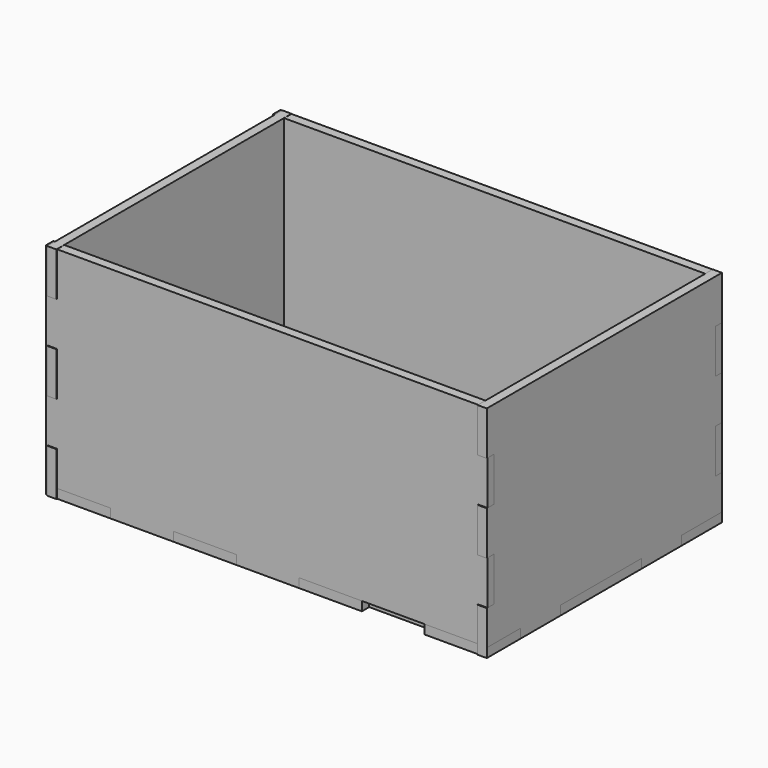
from build123d import *

# Parameters (mm, degrees)
F0_W     = 18.5964285714
F0_H     = 3.175
F0_W_2   = 3.175
F0_H_2   = 14.2994610153
F0_H_3   = 17.4744610153
F0_H_4   = 11.0526949236
F0_W_3   = 21.7714285714
F1_DEPTH = 3.175
F2_W     = 3.175
F2_H     = 15.24
F2_W_2   = 2.8866035402
F3_DEPTH = 3.175
F6_DEPTH = 3.175


with BuildPart() as f1:
    # F0 (on Top) → F1 (new body)
    with BuildSketch(Plane.XY):
        with Locations((-63.7267857143, 49.2125)):
            Rectangle(F0_W, F0_H)
        with Locations((-74.6125, 49.2125)):
            Rectangle(F0_W_2, F0_H)
        with Locations((-74.6125, 40.4752694924)):
            Rectangle(F0_W_2, F0_H_2)
        with Locations((-74.6125, 7.1138474618)):
            Rectangle(F0_W_2, F0_H_3)
        with Locations((-74.6125, -10.3606135535)):
            Rectangle(F0_W_2, F0_H_3)
        with Locations((-74.6125, -42.0986525382)):
            Rectangle(F0_W_2, F0_H_4)
        with Locations((-74.6125, -49.2125)):
            Rectangle(F0_W_2, F0_H)
        with Locations((-63.7267857143, -49.2125)):
            Rectangle(F0_W, F0_H)
        with Locations((-21.7714285714, -49.2125)):
            Rectangle(F0_W_3, F0_H)
        with Locations((21.7714285714, -49.2125)):
            Rectangle(F0_W_3, F0_H)
        with Locations((63.7267857143, -49.2125)):
            Rectangle(F0_W, F0_H)
        with Locations((74.6125, -42.0986525382)):
            Rectangle(F0_W_2, F0_H_4)
        with Locations((74.6125, -10.3606135535)):
            Rectangle(F0_W_2, F0_H_3)
        with Locations((74.6125, 7.1138474618)):
            Rectangle(F0_W_2, F0_H_3)
        with Locations((74.6125, 40.4752694924)):
            Rectangle(F0_W_2, F0_H_2)
        with Locations((74.6125, 49.2125)):
            Rectangle(F0_W_2, F0_H)
        with Locations((63.7267857143, 49.2125)):
            Rectangle(F0_W, F0_H)
        with Locations((21.7714285714, 49.2125)):
            Rectangle(F0_W_3, F0_H)
        with Locations((-21.7714285714, 49.2125)):
            Rectangle(F0_W_3, F0_H)
        Polygon((73.025, 33.3255389847), (73.025, 47.625), (54.4285714286, 47.625), (32.6571428571, 47.625), (10.8857142857, 47.625), (-10.8857142857, 47.625), (-32.6571428571, 47.625), (-54.4285714286, 47.625), (-73.025, 47.625), (-73.025, 33.3255389847), (-73.025, 15.8510779694), (-73.025, -1.6233830458), (-73.025, -19.0978440611), (-73.025, -36.5723050764), (-73.025, -47.625), (-54.4285714286, -47.625), (-32.6571428571, -47.625), (-10.8857142857, -47.625), (10.8857142857, -47.625), (32.6571428571, -47.625), (54.4285714286, -47.625), (73.025, -47.625), (73.025, -36.5723050764), (73.025, -19.0978440611), (73.025, -1.6233830458), (73.025, 15.8510779694), align=None)
    extrude(amount=F1_DEPTH)

    # F2 (on face) → F3 (join)
    with BuildSketch(Plane.YZ.offset(76.2)):
        with Locations((-49.5008964598, 68.58)):
            Rectangle(F2_W, F2_H)
        with Locations((-49.5008964598, 38.1)):
            Rectangle(F2_W, F2_H)
        with Locations((-49.5008964598, 7.62)):
            Rectangle(F2_W, F2_H)
        with Locations((49.3566982299, 38.1)):
            Rectangle(F2_W_2, F2_H)
        with Locations((49.3566982299, 7.62)):
            Rectangle(F2_W_2, F2_H)
        with Locations((49.3566982299, 68.58)):
            Rectangle(F2_W_2, F2_H)
        Polygon((-36.5723050764, 0), (47.9133964598, 0), (47.9133964598, 15.24), (47.9133964598, 30.48), (47.9133964598, 45.72), (47.9133964598, 60.96), (47.9133964598, 76.2), (-47.9133964598, 76.2), (-47.9133964598, 60.96), (-47.9133964598, 45.72), (-47.9133964598, 30.48), (-47.9133964598, 15.24), (-47.9133964598, 0), (-47.625, 0), (-47.625, 3.175), (-36.5723050764, 3.175), align=None)
    extrude(amount=-F3_DEPTH)


with BuildPart() as f4_1:
    # F4: instance of F1
    add(f1.part.mirror(Plane.YZ))


with BuildPart() as f6:
    # F5 (on face) → F6 (new body)
    with BuildSketch(Plane(origin=(0, 47.625, 0), x_dir=(-1, 0, 0), z_dir=(0, 1, 0))):
        Polygon((-76.2, 76.1423557997), (-76.2, 0), (-54.4285714286, 0), (-54.4285714286, 3.175), (-32.6571428571, 3.175), (-32.6571428571, 0), (76.8211558461, 0), (76.8211558461, 76.1423557997), align=None)
    extrude(amount=F6_DEPTH)


with BuildPart() as f7_1:
    # F7: instance of F6
    add(f6.part.mirror(Plane.XZ))

    # F8: cut F1, F4_1
    add(f1.part, mode=Mode.SUBTRACT)
    add(f4_1.part, mode=Mode.SUBTRACT)


with BuildPart() as f6_1:
    add(f6.part)

    # F8: cut F1, F4_1
    add(f1.part, mode=Mode.SUBTRACT)
    add(f4_1.part, mode=Mode.SUBTRACT)


solid = Compound([f1.part, f4_1.part, f7_1.part, f6_1.part])
